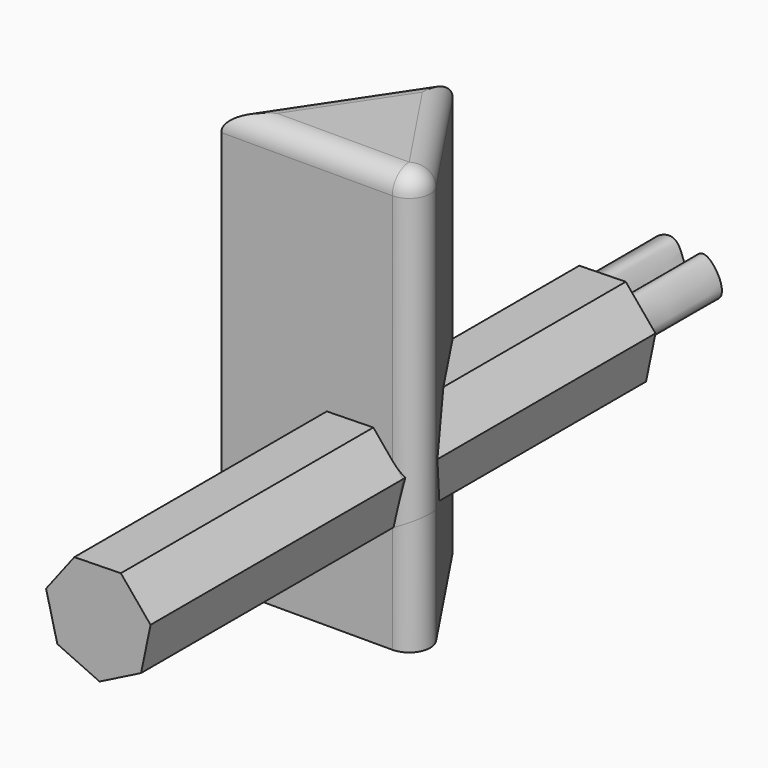
from build123d import *

# Parameters (mm, degrees)
F1_DEPTH     = 50.8
F3_DEPTH     = 76.2
F5_DEPTH     = 25.4
F6_T1_DEPTH  = 48.9984343719
F6_T3_DEPTH  = 71.1905011984
F6_T5_DEPTH  = 54.0079331735
F6_T10_DEPTH = 5.08
F6_T16_DEPTH = 120.2501670661
F6_T22_DEPTH = 120.2501670661
F6_T29_DEPTH = 120.2501670661
F6_T35_DEPTH = 120.2501670661
F6_T42_DEPTH = 120.2501670661
F6_T49_DEPTH = 120.2501670661


# Not quite as in the source:
# - a fillet or chamfer that OpenCascade refuses, or shapes differently, is made with other operations: its cross-section is extruded or revolved along the edge and cut away or added


with BuildPart() as f1:
    # F0 (on Top) → F1 (new body, symmetric)
    with BuildSketch(Plane.XY):
        Polygon((25.4, -38.1), (0, 0), (-25.4, -38.1), align=None)
    extrude(amount=F1_DEPTH, both=True)

    # F2 (on face) → F3 (join, symmetric)
    with BuildSketch(Plane.XZ.offset(38.1)):
        Polygon((0.0813317902, -5.2626694994), (-6.7424972958, -14.1770650191), (-4.0275300761, -25.0701841258), (6.1818077576, -29.739285953), (16.197676584, -24.6684415925), (18.4779228904, -13.6761002742), (11.3054746994, -5.0397192136), align=None)
    extrude(amount=F3_DEPTH, both=True)

    # F4 (on face) → F5 (join)
    with BuildSketch(Plane(origin=(0, 38.1, 0), x_dir=(-1, 0, 0), z_dir=(0, 1, 0))):
        with BuildLine():
            add(Edge.make_bspline(
                [(2.9162010178, -12.9975462332), (1.8670415569, -17.0409513366), (-20.5549326749, -23.97997421), (-9.0441910265, -5.0233845041), (-5.2404331156, -18.2414045319), (-4.2889415012, -5.528991709), (3.5750196715, -10.4584939673), (2.9162010178, -12.9975462332)],
                knots=[0, 0, 0, 0, 0.2848563236, 0.490695137, 0.6535359084, 0.8211247512, 1, 1, 1, 1], degree=3))
        make_face()
    extrude(amount=F5_DEPTH)

    # F6: fillet of radius 5.08 on 4 edges, made by hand

    # F6_s2 → F6_t1 (cut)
    with BuildSketch(Plane(origin=(20.1347486688, -30.2021230032, 0), x_dir=(0, 0, 1), z_dir=(-0.5547001962, 0.8320502943, 0))):
        with BuildLine():
            ThreePointArc((45.72, 0), (49.3121024484, -1.4878975516), (50.8, -5.08))
            Line((50.8, -5.08), (50.8, 0))
            Line((50.8, 0), (45.72, 0))
        make_face()
    extrude(amount=F6_T1_DEPTH, mode=Mode.SUBTRACT)

    # F6_s4 → F6_t3 (cut)
    with BuildSketch(Plane(origin=(7.0446924921, 10.5670387381, 0), x_dir=(0, 0, 1), z_dir=(-0.5547001962, -0.8320502943, 0))):
        with BuildLine():
            ThreePointArc((50.8, -5.08), (49.3121024484, -1.4878975516), (45.72, 0))
            Line((45.72, 0), (50.8, 0))
            Line((50.8, 0), (50.8, -5.08))
        make_face()
    extrude(amount=F6_T3_DEPTH, mode=Mode.SUBTRACT)

    # F6_s6 → F6_t5 (cut)
    with BuildSketch(Plane.YZ.offset(-38.1)):
        with BuildLine():
            ThreePointArc((-38.1, 45.72), (-36.6121024484, 49.3121024484), (-33.02, 50.8))
            Line((-33.02, 50.8), (-38.1, 50.8))
            Line((-38.1, 50.8), (-38.1, 45.72))
        make_face()
    extrude(amount=F6_T5_DEPTH, mode=Mode.SUBTRACT)


with BuildPart() as f6_tool8:
    # F6_s9 → F6_t10 (new body)
    with BuildSketch(Plane.XY.offset(45.72)):
        Polygon((15.9079331735, -33.02), (20.1347486688, -30.2021230032), (25.4, -38.1), (15.9079331735, -38.1), align=None)
    extrude(amount=F6_T10_DEPTH)

    # F6_s11 → F6_t12 (revolve, cut)
    with BuildSketch(Plane(origin=(15.9079331735, -33.02, 45.72), x_dir=(-0.8816745988, 0.4718579255, 0), z_dir=(0.4718579255, 0.8816745988, 0))):
        with BuildLine():
            ThreePointArc((0, -5.08), (5.08, 0), (0, 5.08))
            Line((0, 5.08), (0, -5.08))
        make_face()
    revolve(axis=Axis((15.9079331735, -33.02, 45.72), (0, 0, 1)), mode=Mode.SUBTRACT)


with BuildPart() as f1_1:
    add(f1.part)

    # F6_t7: cut F6_tool8
    add(f6_tool8.part, mode=Mode.SUBTRACT)


with BuildPart() as f6_tool14:
    # F6_s15 → F6_t16 (new body)
    with BuildSketch(Plane.XY.offset(45.72)):
        with BuildLine():
            ThreePointArc((20.1347486688, -30.2021230032), (20.3868401353, -35.4170382617), (15.9079331735, -38.1))
            Line((15.9079331735, -38.1), (25.4, -38.1))
            Line((25.4, -38.1), (20.1347486688, -30.2021230032))
        make_face()
    extrude(amount=-F6_T16_DEPTH)

    split(bisect_by=Plane(origin=(20.4355225798, 0, -4.2391355518), x_dir=(0, 1, 0), z_dir=(-0.9791548002, 0, 0.2031154284)), keep=Keep.TOP)

    split(bisect_by=Plane(origin=(4.2137378339, 0, 3.4994769327), x_dir=(0, 1, 0), z_dir=(0.7692950689, 0, 0.6388936508)), keep=Keep.TOP)


with BuildPart() as f1_2:
    add(f1_1.part)

    # F6_t13: cut F6_tool14
    add(f6_tool14.part, mode=Mode.SUBTRACT)


with BuildPart() as f6_tool20:
    # F6_s21 → F6_t22 (new body)
    with BuildSketch(Plane.XY.offset(45.72)):
        with BuildLine():
            ThreePointArc((20.1347486688, -30.2021230032), (20.3868401353, -35.4170382617), (15.9079331735, -38.1))
            Line((15.9079331735, -38.1), (25.4, -38.1))
            Line((25.4, -38.1), (20.1347486688, -30.2021230032))
        make_face()
    extrude(amount=-F6_T22_DEPTH)

    split(bisect_by=Plane(origin=(13.2457923387, 0, -26.1629245812), x_dir=(0, 1, 0), z_dir=(-0.4516909958, 0, 0.8921744472)), keep=Keep.TOP)

    split(bisect_by=Plane(origin=(20.4355225798, 0, -4.2391355518), x_dir=(0, 1, 0), z_dir=(0.9791548002, 0, -0.2031154284)), keep=Keep.TOP)

    split(bisect_by=Plane(origin=(4.2137378339, 0, 3.4994769327), x_dir=(0, 1, 0), z_dir=(0.7692950689, 0, 0.6388936508)), keep=Keep.TOP)


with BuildPart() as f1_3:
    add(f1_2.part)

    # F6_t19: cut F6_tool20
    add(f6_tool20.part, mode=Mode.SUBTRACT)


with BuildPart() as f6_tool27:
    # F6_s28 → F6_t29 (new body)
    with BuildSketch(Plane.XY.offset(45.72)):
        with BuildLine():
            ThreePointArc((20.1347486688, -30.2021230032), (20.3868401353, -35.4170382617), (15.9079331735, -38.1))
            Line((15.9079331735, -38.1), (25.4, -38.1))
            Line((25.4, -38.1), (20.1347486688, -30.2021230032))
        make_face()
    extrude(amount=-F6_T29_DEPTH)

    split(bisect_by=Plane(origin=(13.2457923387, 0, -26.1629245812), x_dir=(0, 1, 0), z_dir=(0.4516909958, 0, -0.8921744472)), keep=Keep.TOP)

    split(bisect_by=Plane(origin=(20.4355225798, 0, -4.2391355518), x_dir=(0, 1, 0), z_dir=(-0.9791548002, 0, 0.2031154284)), keep=Keep.TOP)


with BuildPart() as f1_4:
    add(f1_3.part)

    # F6_t26: cut F6_tool27
    add(f6_tool27.part, mode=Mode.SUBTRACT)


with BuildPart() as f6_tool33:
    # F6_s34 → F6_t35 (new body)
    with BuildSketch(Plane.XY.offset(45.72)):
        with BuildLine():
            ThreePointArc((20.1347486688, -30.2021230032), (20.3868401353, -35.4170382617), (15.9079331735, -38.1))
            Line((15.9079331735, -38.1), (25.4, -38.1))
            Line((25.4, -38.1), (20.1347486688, -30.2021230032))
        make_face()
    extrude(amount=-F6_T35_DEPTH)

    split(bisect_by=Plane(origin=(13.2457923387, 0, -26.1629245812), x_dir=(0, 1, 0), z_dir=(-0.4516909958, 0, 0.8921744472)), keep=Keep.TOP)

    split(bisect_by=Plane(origin=(20.4355225798, 0, -4.2391355518), x_dir=(0, 1, 0), z_dir=(0.9791548002, 0, -0.2031154284)), keep=Keep.TOP)

    split(bisect_by=Plane(origin=(4.2137378339, 0, 3.4994769327), x_dir=(0, 1, 0), z_dir=(-0.7692950689, 0, -0.6388936508)), keep=Keep.TOP)


with BuildPart() as f1_5:
    add(f1_4.part)

    # F6_t32: cut F6_tool33
    add(f6_tool33.part, mode=Mode.SUBTRACT)


with BuildPart() as f6_tool40:
    # F6_s41 → F6_t42 (new body)
    with BuildSketch(Plane.XY.offset(45.72)):
        with BuildLine():
            ThreePointArc((20.1347486688, -30.2021230032), (20.3868401353, -35.4170382617), (15.9079331735, -38.1))
            Line((15.9079331735, -38.1), (25.4, -38.1))
            Line((25.4, -38.1), (20.1347486688, -30.2021230032))
        make_face()
    extrude(amount=-F6_T42_DEPTH)

    split(bisect_by=Plane(origin=(13.2457923387, 0, -26.1629245812), x_dir=(0, 1, 0), z_dir=(0.4516909958, 0, -0.8921744472)), keep=Keep.TOP)

    split(bisect_by=Plane(origin=(20.4355225798, 0, -4.2391355518), x_dir=(0, 1, 0), z_dir=(0.9791548002, 0, -0.2031154284)), keep=Keep.TOP)

    split(bisect_by=Plane(origin=(4.2137378339, 0, 3.4994769327), x_dir=(0, 1, 0), z_dir=(-0.7692950689, 0, -0.6388936508)), keep=Keep.TOP)


with BuildPart() as f1_6:
    add(f1_5.part)

    # F6_t39: cut F6_tool40
    add(f6_tool40.part, mode=Mode.SUBTRACT)


with BuildPart() as f6_tool47:
    # F6_s48 → F6_t49 (new body)
    with BuildSketch(Plane.XY.offset(45.72)):
        with BuildLine():
            ThreePointArc((20.1347486688, -30.2021230032), (20.3868401353, -35.4170382617), (15.9079331735, -38.1))
            Line((15.9079331735, -38.1), (25.4, -38.1))
            Line((25.4, -38.1), (20.1347486688, -30.2021230032))
        make_face()
    extrude(amount=-F6_T49_DEPTH)

    split(bisect_by=Plane(origin=(13.2457923387, 0, -26.1629245812), x_dir=(0, 1, 0), z_dir=(0.4516909958, 0, -0.8921744472)), keep=Keep.TOP)

    split(bisect_by=Plane(origin=(4.2137378339, 0, 3.4994769327), x_dir=(0, 1, 0), z_dir=(0.7692950689, 0, 0.6388936508)), keep=Keep.TOP)


with BuildPart() as f1_7:
    add(f1_6.part)

    # F6_t46: cut F6_tool47
    add(f6_tool47.part, mode=Mode.SUBTRACT)


solid = f1_7.part
